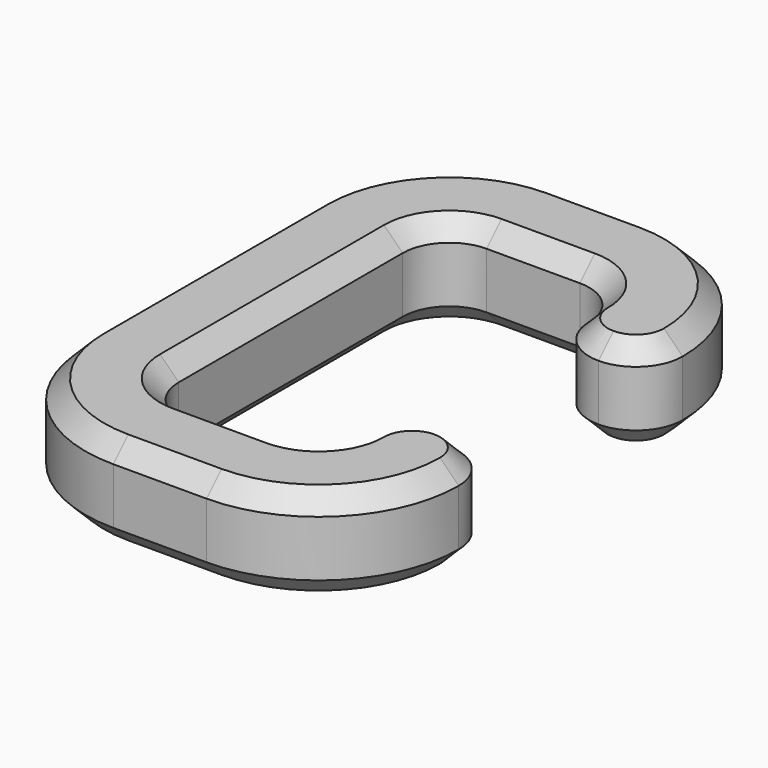
from build123d import *

# Parameters (mm, degrees)
F0_W         = 10
F0_H         = 10
F1_DEPTH     = 10
F2_R         = 4.99999
F3_R         = 15
F4_T1_DEPTH  = 30
F4_T3_DEPTH  = 10
F4_T5_DEPTH  = 1e-05
F4_T7_DEPTH  = 2e-05
F4_T9_DEPTH  = 2e-05
F4_T11_DEPTH = 10.00002
F4_T13_DEPTH = 30.00002
F4_T15_DEPTH = 2e-05
F4_T17_DEPTH = 1e-05
F4_T20_ANGLE = 90
F4_T22_ANGLE = 90
F4_T24_ANGLE = 90
F4_T26_ANGLE = 90
F4_T28_ANGLE = 90
F4_T30_ANGLE = 90
F4_T32_ANGLE = 90
F4_T34_ANGLE = 90
F4_T36_ANGLE = 90
F4_T38_ANGLE = 90
F4_T40_ANGLE = 90
F4_T42_ANGLE = 90
F4_T44_ANGLE = 90
F4_T46_ANGLE = 90
F4_T48_ANGLE = 90
F4_T50_ANGLE = 90
F4_T52_ANGLE = 90
F4_T54_ANGLE = 90
F4_T56_ANGLE = 90
F4_T58_ANGLE = 90
F4_T60_ANGLE = 90
F4_T62_ANGLE = 90
F4_T64_ANGLE = 90
F4_T66_ANGLE = 90


# Not quite as in the source:
# - a fillet or chamfer that OpenCascade refuses, or shapes differently, is made with other operations: its cross-section is extruded or revolved along the edge and cut away or added
# - a fillet or chamfer is up to 0.001 mm smaller than in the source, because OpenCascade refuses the exact size


with BuildPart() as f1:
    # F0 (on Top) → F1 (new body)
    with BuildSketch(Plane.XY):
        Polygon((-4.4905686265, 20.6948744461), (-34.4905686265, 20.6948744461), (-34.4905686265, 10.6948744461), (-24.4905686265, 10.6948744461), (-4.4905686265, 10.6948744461), align=None)
        Polygon((5.5094313735, 20.6948744461), (-4.4905686265, 20.6948744461), (-4.4905686265, 10.6948744461), (-4.4905686265, 0.6948744461), (5.5094313735, 0.6948744461), align=None)
        with Locations((0.5094313735, -24.3051255539)):
            Rectangle(F0_W, F0_H)
        Polygon((-24.4905686265, 10.6948744461), (-34.4905686265, 10.6948744461), (-34.4905686265, -39.3051255539), (-24.4905686265, -39.3051255539), (-24.4905686265, -29.3051255539), align=None)
        Polygon((-4.4905686265, -29.3051255539), (-24.4905686265, -29.3051255539), (-24.4905686265, -39.3051255539), (5.5094313735, -39.3051255539), (5.5094313735, -29.3051255539), align=None)
    extrude(amount=F1_DEPTH)

    # F2 (radius 5 in the source; OpenCascade refuses exactly that, so slightly less here)
    f2_edges = [f1.edges().sort_by_distance(p)[0] for p in [
        (5.509431, 0.694874, 5),
        (-4.490569, 0.694874, 5),
        (-4.490569, 10.694874, 5),
        (5.509431, -19.305126, 5),
        (-4.490569, -19.305126, 5),
        (-24.490569, 10.694874, 5),
        (-24.490569, -29.305126, 5),
        (-4.490569, -29.305126, 5),
    ]]
    fillet(f2_edges, radius=F2_R)

    # F3
    f3_edges = [f1.edges().sort_by_distance(p)[0] for p in [
        (-34.490569, 20.694874, 5),
        (5.509431, 20.694874, 5),
        (5.509431, -39.305126, 5),
        (-34.490569, -39.305126, 5),
    ]]
    fillet(f3_edges, radius=F3_R)

    # F4: chamfer of 2 on 2 edges, made by hand

    # F4_s2 → F4_t1 (cut)
    with BuildSketch(Plane.XZ.offset(-5.6948744461)):
        Polygon((-32.4905686265, 10), (-34.4905686265, 8), (-34.4905686265, 10), align=None)
        Polygon((-32.4905686265, 0), (-34.4905686265, 2), (-34.4905686265, 0), align=None)
    extrude(amount=F4_T1_DEPTH, mode=Mode.SUBTRACT)

    # F4_s4 → F4_t3 (cut)
    with BuildSketch(Plane.YZ.offset(-19.4905686265)):
        Polygon((-37.3051255539, 0), (-39.3051255539, 2), (-39.3051255539, 0), align=None)
        Polygon((18.6948744461, 0), (20.6948744461, 2), (20.6948744461, 0), align=None)
        Polygon((-37.3051255539, 10), (-39.3051255539, 8), (-39.3051255539, 10), align=None)
        Polygon((18.6948744461, 10), (20.6948744461, 8), (20.6948744461, 10), align=None)
    extrude(amount=F4_T3_DEPTH, mode=Mode.SUBTRACT)

    # F4_s6 → F4_t5 (cut)
    with BuildSketch(Plane.XZ.offset(24.3051155539)):
        Polygon((5.5094313735, 2), (3.5094313735, 0), (5.5094313735, 0), align=None)
        Polygon((5.5094313735, 8), (3.5094313735, 10), (5.5094313735, 10), align=None)
    extrude(amount=F4_T5_DEPTH, mode=Mode.SUBTRACT)

    # F4_s8 → F4_t7 (cut)
    with BuildSketch(Plane.YZ.offset(0.5094213735)):
        Polygon((-21.3051255539, 0), (-19.3051255539, 2), (-19.3051255539, 0), align=None)
        Polygon((2.6948744461, 0), (0.6948744461, 2), (0.6948744461, 0), align=None)
        Polygon((-21.3051255539, 10), (-19.3051255539, 8), (-19.3051255539, 10), align=None)
        Polygon((2.6948744461, 10), (0.6948744461, 8), (0.6948744461, 10), align=None)
    extrude(amount=F4_T7_DEPTH, mode=Mode.SUBTRACT)

    # F4_s10 → F4_t9 (cut)
    with BuildSketch(Plane.XZ.offset(24.3051155539)):
        Polygon((-2.4905686265, 0), (-4.4905686265, 2), (-4.4905686265, 0), align=None)
        Polygon((-2.4905686265, 10), (-4.4905686265, 8), (-4.4905686265, 10), align=None)
    extrude(amount=F4_T9_DEPTH, mode=Mode.SUBTRACT)

    # F4_s12 → F4_t11 (cut)
    with BuildSketch(Plane.YZ.offset(-19.4905786265)):
        Polygon((-31.3051255539, 0), (-29.3051255539, 2), (-29.3051255539, 0), align=None)
        Polygon((12.6948744461, 0), (10.6948744461, 2), (10.6948744461, 0), align=None)
        Polygon((-31.3051255539, 10), (-29.3051255539, 8), (-29.3051255539, 10), align=None)
        Polygon((12.6948744461, 10), (10.6948744461, 8), (10.6948744461, 10), align=None)
    extrude(amount=F4_T11_DEPTH, mode=Mode.SUBTRACT)

    # F4_s14 → F4_t13 (cut)
    with BuildSketch(Plane.XZ.offset(-5.6948844461)):
        Polygon((-26.4905686265, 0), (-24.4905686265, 2), (-24.4905686265, 0), align=None)
        Polygon((-26.4905686265, 10), (-24.4905686265, 8), (-24.4905686265, 10), align=None)
    extrude(amount=F4_T13_DEPTH, mode=Mode.SUBTRACT)

    # F4_s16 → F4_t15 (cut)
    with BuildSketch(Plane.XZ.offset(-5.6948844461)):
        Polygon((-2.4905686265, 0), (-4.4905686265, 2), (-4.4905686265, 0), align=None)
        Polygon((-2.4905686265, 10), (-4.4905686265, 8), (-4.4905686265, 10), align=None)
    extrude(amount=F4_T15_DEPTH, mode=Mode.SUBTRACT)

    # F4_s18 → F4_t17 (cut)
    with BuildSketch(Plane.XZ.offset(-5.6948744461)):
        Polygon((3.5094313735, 0), (5.5094313735, 2), (5.5094313735, 0), align=None)
        Polygon((3.5094313735, 10), (5.5094313735, 8), (5.5094313735, 10), align=None)
    extrude(amount=F4_T17_DEPTH, mode=Mode.SUBTRACT)

    # F4_s19 → F4_t20 (revolve, cut)
    with BuildSketch(Plane.XZ.offset(-5.6948744461)):
        Polygon((-32.4905686265, 0), (-34.4905686265, 2), (-34.4905686265, 0), align=None)
    revolve(axis=Axis((-19.4905686265, 5.6948744461, 0), (0, 0, -1)), revolution_arc=F4_T20_ANGLE, mode=Mode.SUBTRACT)

    # F4_s21 → F4_t22 (revolve, cut)
    with BuildSketch(Plane.YZ.offset(-19.4905686265)):
        Polygon((-37.3051255539, 0), (-39.3051255539, 2), (-39.3051255539, 0), align=None)
    revolve(axis=Axis((-19.4905686265, -24.3051255539, 0), (0, 0, -1)), revolution_arc=F4_T22_ANGLE, mode=Mode.SUBTRACT)

    # F4_s23 → F4_t24 (revolve, cut)
    with BuildSketch(Plane.XZ.offset(24.3051255539)):
        Polygon((3.5094313735, 0), (5.5094313735, 2), (5.5094313735, 0), align=None)
    revolve(axis=Axis((-9.4905686265, -24.3051255539, 0), (0, 0, -1)), revolution_arc=F4_T24_ANGLE, mode=Mode.SUBTRACT)

    # F4_s25 → F4_t26 (revolve, cut)
    with BuildSketch(Plane.XZ.offset(24.3051155539)):
        Polygon((3.5094313735, 0), (5.5094313735, 2), (5.5094313735, 0), align=None)
    revolve(axis=Axis((0.5094413735, -24.3051155539, 0), (0, 0, 1)), revolution_arc=F4_T26_ANGLE, mode=Mode.SUBTRACT)

    # F4_s27 → F4_t28 (revolve, cut)
    with BuildSketch(Plane.YZ.offset(0.5094213735)):
        Polygon((-21.3051255539, 0), (-19.3051255539, 2), (-19.3051255539, 0), align=None)
    revolve(axis=Axis((0.5094213735, -24.3051155539, 0), (0, 0, 1)), revolution_arc=F4_T28_ANGLE, mode=Mode.SUBTRACT)

    # F4_s29 → F4_t30 (revolve, cut)
    with BuildSketch(Plane.XZ.offset(24.3051355539)):
        Polygon((-2.4905686265, 0), (-4.4905686265, 2), (-4.4905686265, 0), align=None)
    revolve(axis=Axis((-9.4905586265, -24.3051355539, 0), (0, 0, -1)), revolution_arc=F4_T30_ANGLE, mode=Mode.SUBTRACT)

    # F4_s31 → F4_t32 (revolve, cut)
    with BuildSketch(Plane.YZ.offset(-19.4905786265)):
        Polygon((-31.3051255539, 0), (-29.3051255539, 2), (-29.3051255539, 0), align=None)
    revolve(axis=Axis((-19.4905786265, -24.3051355539, 0), (0, 0, -1)), revolution_arc=F4_T32_ANGLE, mode=Mode.SUBTRACT)

    # F4_s33 → F4_t34 (revolve, cut)
    with BuildSketch(Plane.XZ.offset(-5.6948844461)):
        Polygon((-26.4905686265, 0), (-24.4905686265, 2), (-24.4905686265, 0), align=None)
    revolve(axis=Axis((-19.4905786265, 5.6948844461, 0), (0, 0, -1)), revolution_arc=F4_T34_ANGLE, mode=Mode.SUBTRACT)

    # F4_s35 → F4_t36 (revolve, cut)
    with BuildSketch(Plane.YZ.offset(-9.4905586265)):
        Polygon((12.6948744461, 0), (10.6948744461, 2), (10.6948744461, 0), align=None)
    revolve(axis=Axis((-9.4905586265, 5.6948844461, 0), (0, 0, -1)), revolution_arc=F4_T36_ANGLE, mode=Mode.SUBTRACT)

    # F4_s37 → F4_t38 (revolve, cut)
    with BuildSketch(Plane.XZ.offset(-5.6948644461)):
        Polygon((-2.4905686265, 0), (-4.4905686265, 2), (-4.4905686265, 0), align=None)
    revolve(axis=Axis((0.5094213735, 5.6948644461, 0), (0, 0, 1)), revolution_arc=F4_T38_ANGLE, mode=Mode.SUBTRACT)

    # F4_s39 → F4_t40 (revolve, cut)
    with BuildSketch(Plane.YZ.offset(0.5094413735)):
        Polygon((2.6948744461, 0), (0.6948744461, 2), (0.6948744461, 0), align=None)
    revolve(axis=Axis((0.5094413735, 5.6948644461, 0), (0, 0, 1)), revolution_arc=F4_T40_ANGLE, mode=Mode.SUBTRACT)

    # F4_s41 → F4_t42 (revolve, cut)
    with BuildSketch(Plane.YZ.offset(-9.4905686265)):
        Polygon((18.6948744461, 0), (20.6948744461, 2), (20.6948744461, 0), align=None)
    revolve(axis=Axis((-9.4905686265, 5.6948744461, 0), (0, 0, -1)), revolution_arc=F4_T42_ANGLE, mode=Mode.SUBTRACT)

    # F4_s43 → F4_t44 (revolve, cut)
    with BuildSketch(Plane.XZ.offset(-5.6948744461)):
        Polygon((-32.4905686265, 10), (-34.4905686265, 8), (-34.4905686265, 10), align=None)
    revolve(axis=Axis((-19.4905686265, 5.6948744461, 10), (0, 0, -1)), revolution_arc=F4_T44_ANGLE, mode=Mode.SUBTRACT)

    # F4_s45 → F4_t46 (revolve, cut)
    with BuildSketch(Plane.YZ.offset(-19.4905686265)):
        Polygon((-37.3051255539, 10), (-39.3051255539, 8), (-39.3051255539, 10), align=None)
    revolve(axis=Axis((-19.4905686265, -24.3051255539, 10), (0, 0, -1)), revolution_arc=F4_T46_ANGLE, mode=Mode.SUBTRACT)

    # F4_s47 → F4_t48 (revolve, cut)
    with BuildSketch(Plane.XZ.offset(24.3051255539)):
        Polygon((5.5094313735, 8), (3.5094313735, 10), (5.5094313735, 10), align=None)
    revolve(axis=Axis((-9.4905686265, -24.3051255539, 10), (0, 0, -1)), revolution_arc=F4_T48_ANGLE, mode=Mode.SUBTRACT)

    # F4_s49 → F4_t50 (revolve, cut)
    with BuildSketch(Plane.XZ.offset(24.3051155539)):
        Polygon((5.5094313735, 8), (3.5094313735, 10), (5.5094313735, 10), align=None)
    revolve(axis=Axis((0.5094413735, -24.3051155539, 10), (0, 0, 1)), revolution_arc=F4_T50_ANGLE, mode=Mode.SUBTRACT)

    # F4_s51 → F4_t52 (revolve, cut)
    with BuildSketch(Plane.YZ.offset(0.5094213735)):
        Polygon((-21.3051255539, 10), (-19.3051255539, 8), (-19.3051255539, 10), align=None)
    revolve(axis=Axis((0.5094213735, -24.3051155539, 10), (0, 0, 1)), revolution_arc=F4_T52_ANGLE, mode=Mode.SUBTRACT)

    # F4_s53 → F4_t54 (revolve, cut)
    with BuildSketch(Plane.XZ.offset(24.3051355539)):
        Polygon((-2.4905686265, 10), (-4.4905686265, 8), (-4.4905686265, 10), align=None)
    revolve(axis=Axis((-9.4905586265, -24.3051355539, 10), (0, 0, -1)), revolution_arc=F4_T54_ANGLE, mode=Mode.SUBTRACT)

    # F4_s55 → F4_t56 (revolve, cut)
    with BuildSketch(Plane.YZ.offset(-19.4905786265)):
        Polygon((-31.3051255539, 10), (-29.3051255539, 8), (-29.3051255539, 10), align=None)
    revolve(axis=Axis((-19.4905786265, -24.3051355539, 10), (0, 0, -1)), revolution_arc=F4_T56_ANGLE, mode=Mode.SUBTRACT)

    # F4_s57 → F4_t58 (revolve, cut)
    with BuildSketch(Plane.XZ.offset(-5.6948844461)):
        Polygon((-26.4905686265, 10), (-24.4905686265, 8), (-24.4905686265, 10), align=None)
    revolve(axis=Axis((-19.4905786265, 5.6948844461, 10), (0, 0, -1)), revolution_arc=F4_T58_ANGLE, mode=Mode.SUBTRACT)

    # F4_s59 → F4_t60 (revolve, cut)
    with BuildSketch(Plane.YZ.offset(-9.4905586265)):
        Polygon((12.6948744461, 10), (10.6948744461, 8), (10.6948744461, 10), align=None)
    revolve(axis=Axis((-9.4905586265, 5.6948844461, 10), (0, 0, -1)), revolution_arc=F4_T60_ANGLE, mode=Mode.SUBTRACT)

    # F4_s61 → F4_t62 (revolve, cut)
    with BuildSketch(Plane.XZ.offset(-5.6948644461)):
        Polygon((-2.4905686265, 10), (-4.4905686265, 8), (-4.4905686265, 10), align=None)
    revolve(axis=Axis((0.5094213735, 5.6948644461, 10), (0, 0, 1)), revolution_arc=F4_T62_ANGLE, mode=Mode.SUBTRACT)

    # F4_s63 → F4_t64 (revolve, cut)
    with BuildSketch(Plane.YZ.offset(0.5094413735)):
        Polygon((2.6948744461, 10), (0.6948744461, 8), (0.6948744461, 10), align=None)
    revolve(axis=Axis((0.5094413735, 5.6948644461, 10), (0, 0, 1)), revolution_arc=F4_T64_ANGLE, mode=Mode.SUBTRACT)

    # F4_s65 → F4_t66 (revolve, cut)
    with BuildSketch(Plane.YZ.offset(-9.4905686265)):
        Polygon((18.6948744461, 10), (20.6948744461, 8), (20.6948744461, 10), align=None)
    revolve(axis=Axis((-9.4905686265, 5.6948744461, 10), (0, 0, -1)), revolution_arc=F4_T66_ANGLE, mode=Mode.SUBTRACT)


solid = f1.part
